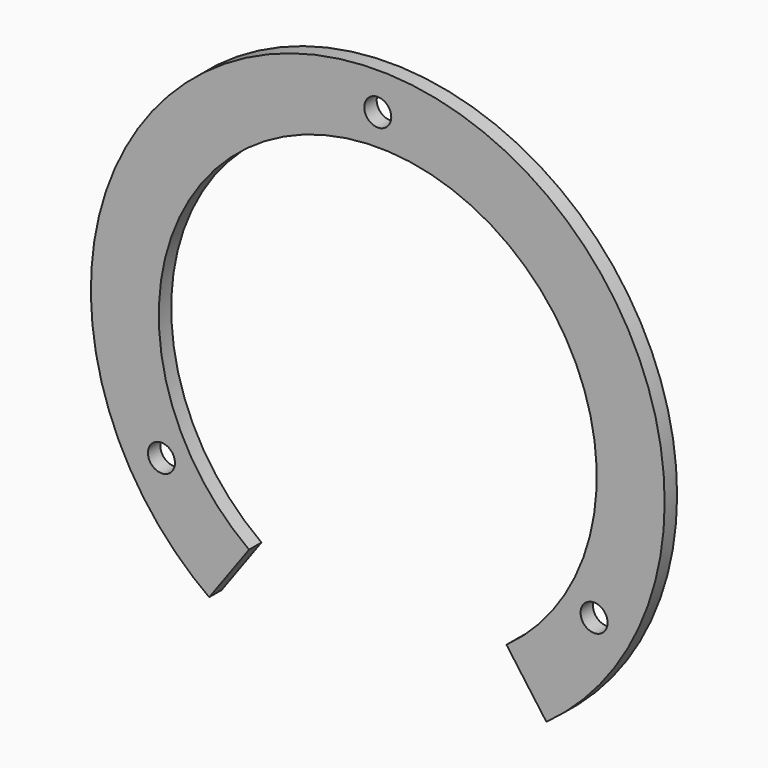
from build123d import *

# Parameters (mm, degrees)
F0_R     = 8
F1_DEPTH = 9.2


with BuildPart() as f1:
    # F0 (on Front) → F1 (new body)
    with BuildSketch(Plane.XZ):
        with BuildLine():
            Line((76.2651364849, -104.9699550201), (99.9234928897, -137.5328890437))
            ThreePointArc((99.9234928897, -137.5328890437), (5.9329144394, 169.8964405932), (-109.2738936467, -130.2275553302))
            Line((-109.2738936467, -130.2275553302), (-99.8627523041, -137.4492867999))
            Line((-99.8627523041, -137.4492867999), (-76.2651364849, -104.9699550201))
            ThreePointArc((-76.2651364849, -104.9699550201), (-10.7051286377, 129.3076282392), (92.4890377243, -90.9991230773))
            ThreePointArc((92.4890377243, -90.9991230773), (84.6657478828, -98.3197520107), (76.2651364849, -104.9699550201))
        make_face()
        with Locations((-128.1717597601, -74)):
            Circle(F0_R, mode=Mode.SUBTRACT)
        with Locations((128.1717597601, -74)):
            Circle(F0_R, mode=Mode.SUBTRACT)
        with Locations((0, 148)):
            Circle(F0_R, mode=Mode.SUBTRACT)
    extrude(amount=F1_DEPTH)


solid = f1.part
